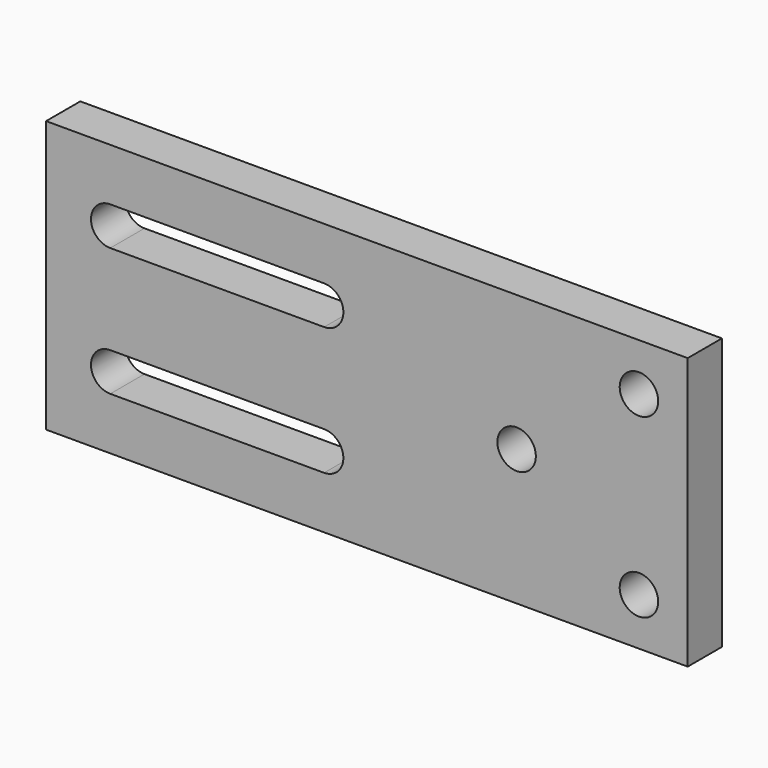
from build123d import *

# Parameters (mm, degrees)
F0_W     = 150
F0_H     = 63.5
F1_DEPTH = 5
F3_DEPTH = 10.001
F5_D     = 9
F5_DEPTH = 18
F5_TIP   = 2.7038727856


with BuildPart() as f1:
    # F0 (on Front) → F1 (new body, symmetric)
    with BuildSketch(Plane.XZ):
        Rectangle(F0_W, F0_H)
    extrude(amount=F1_DEPTH, both=True)

    # F2 (on face) → F3 (cut, through all)
    with BuildSketch(Plane.XZ.offset(5)):
        with BuildLine():
            ThreePointArc((-60, 19.5), (-64.5, 15), (-60, 10.5))
            Line((-60, 10.5), (-10, 10.5))
            ThreePointArc((-10, 10.5), (-5.5, 15), (-10, 19.5))
            Line((-10, 19.5), (-60, 19.5))
        make_face()
        with BuildLine():
            ThreePointArc((-60, -10.5), (-64.5, -15), (-60, -19.5))
            Line((-60, -19.5), (-10, -19.5))
            ThreePointArc((-10, -19.5), (-5.5, -15), (-10, -10.5))
            Line((-10, -10.5), (-60, -10.5))
        make_face()
    extrude(amount=-F3_DEPTH, mode=Mode.SUBTRACT)

    # F5
    with Locations(Plane.XZ.offset(5)):
        with Locations((35, 0), (63.6, 20.65), (63.6, -20.65)):
            Hole(F5_D / 2, depth=F5_DEPTH)
            with Locations((0, 0, -(F5_DEPTH + F5_TIP / 2))):  # 118° drill point
                Cone(0, F5_D / 2, F5_TIP, mode=Mode.SUBTRACT)


solid = f1.part
